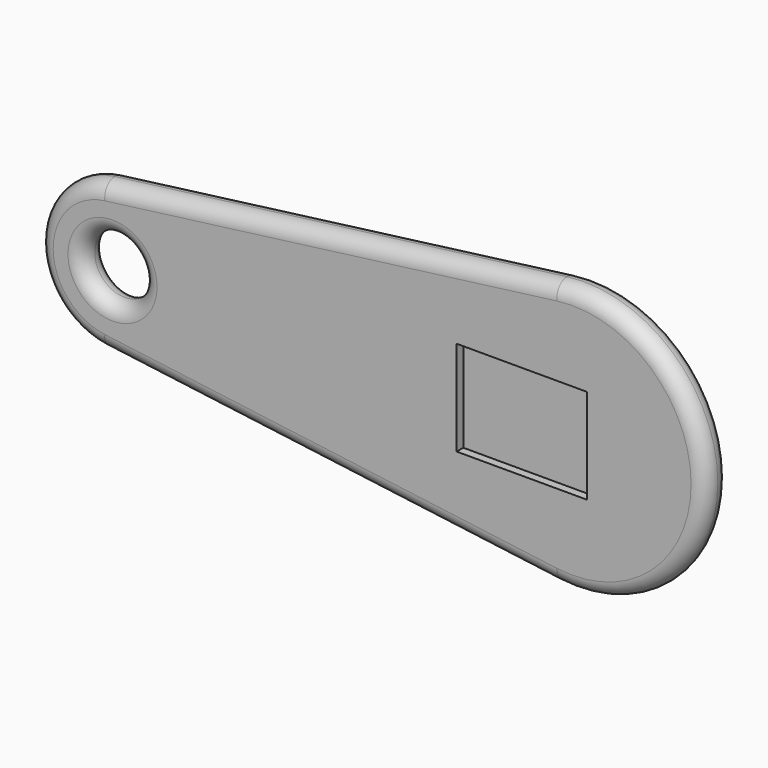
from build123d import *

# Parameters (mm, degrees)
F1_DEPTH = 1.27
F2_R     = 2.54
F3_DEPTH = 25.4
F4_R     = 1.26999
F5_W     = 11.176
F5_H     = 8.128
F6_DEPTH = 0.7112


# Not quite as in the source:
# - a fillet or chamfer is up to 0.001 mm smaller than in the source, because OpenCascade refuses the exact size


with BuildPart() as f1:
    # F0 (on Front) → F1 (new body, symmetric)
    with BuildSketch(Plane.XZ):
        with BuildLine():
            ThreePointArc((-23.6793548387, -6.2969165191), (-18.6695586883, -4.7710273121), (-16.51, 0))
            ThreePointArc((-16.51, 0), (-18.6695586883, 4.7710273121), (-23.6793548387, 6.2969165191))
            ThreePointArc((-23.6793548387, 6.2969165191), (-29.21, 0), (-23.6793548387, -6.2969165191))
        make_face()
        with BuildLine():
            ThreePointArc((-23.6793548387, 6.2969165191), (-18.6695586883, 4.7710273121), (-16.51, 0))
            ThreePointArc((-16.51, 0), (-18.6695586883, -4.7710273121), (-23.6793548387, -6.2969165191))
            Line((-23.6793548387, -6.2969165191), (15.0351612903, -11.3344497343))
            ThreePointArc((15.0351612903, -11.3344497343), (5.08, 0), (15.0351612903, 11.3344497343))
            Line((15.0351612903, 11.3344497343), (-23.6793548387, 6.2969165191))
        make_face()
        with BuildLine():
            ThreePointArc((27.94, 0), (24.0527943611, 8.5878491618), (15.0351612903, 11.3344497343))
            ThreePointArc((15.0351612903, 11.3344497343), (5.08, 0), (15.0351612903, -11.3344497343))
            ThreePointArc((15.0351612903, -11.3344497343), (24.0527943611, -8.5878491618), (27.94, 0))
        make_face()
    extrude(amount=F1_DEPTH, both=True)

    # F2 (on face) → F3 (cut, symmetric)
    with BuildSketch(Plane.XZ.offset(1.27)):
        with Locations((-22.86, 0)):
            Circle(F2_R)
    extrude(amount=F3_DEPTH, both=True, mode=Mode.SUBTRACT)

    # F4 (radius 1.27 in the source; OpenCascade refuses exactly that, so slightly less here)
    f4_edges = [f1.edges().sort_by_distance(p)[0] for p in [
        (-4.322097, -1.27, 8.815683),
        (-4.322097, 1.27, 8.815683),
        (27.94, -1.27, 0),
        (15.035161, 0, -11.33445),
        (27.94, 1.27, 0),
        (15.035161, 0, 11.33445),
        (-29.21, -1.27, 0),
        (-25.4, 1.27, 0),
        (-25.4, -1.27, 0),
        (-29.21, 1.27, 0),
    ]]
    fillet(f4_edges, radius=F4_R)

    # F5 (on face) → F6 (cut)
    with BuildSketch(Plane.XZ.offset(1.27)):
        with Locations((12.192, -0.0039664305)):
            Rectangle(F5_W, F5_H)
    extrude(amount=-F6_DEPTH, mode=Mode.SUBTRACT)


solid = f1.part
